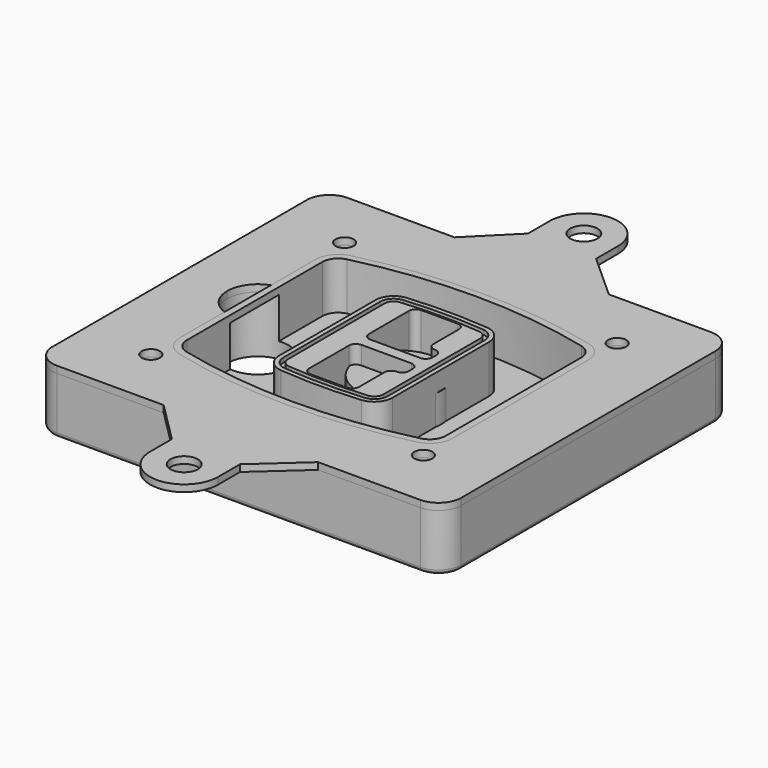
from build123d import *

# Parameters (mm, degrees)
F0_R      = 4
F1_DEPTH  = 25
F2_DEPTH  = 3
F3_DEPTH  = 18
F5_DEPTH  = 21
F6_DEPTH  = 2
F8_DEPTH  = 20
F9_DEPTH  = 16
F10_DEPTH = 25
F7_R      = 6
F7_R_2    = 4
F11_DEPTH = 6
F13_DEPTH = 9
F15_R     = 2
F16_R     = 4
F16_R_2   = 6
F17_DEPTH = 3


# Not quite as in the source:
# - a feature of the source that left no trace in its solid (it failed there, or was rolled back) is left out
# - a feature names something its author has since deleted; it is built from what else it names


with BuildPart() as f1:
    # F0 (on Top) → F1 (new body)
    with BuildSketch(Plane.XY):
        with BuildLine():
            ThreePointArc((-90, -70), (-87.0710678119, -77.0710678119), (-80, -80))
            Line((-80, -80), (80, -80))
            ThreePointArc((80, -80), (87.0710678119, -77.0710678119), (90, -70))
            Line((90, -70), (90, 70))
            ThreePointArc((90, 70), (87.0710678119, 77.0710678119), (80, 80))
            Line((80, 80), (-80, 80))
            ThreePointArc((-80, 80), (-87.0710678119, 77.0710678119), (-90, 70))
            Line((-90, 70), (-90, -70))
        make_face()
        with Locations((-60, -53.3333333333)):
            Circle(F0_R, mode=Mode.SUBTRACT)
        with Locations((60, -53.3333333333)):
            Circle(F0_R, mode=Mode.SUBTRACT)
        with Locations((-60, 53.3333333333)):
            Circle(F0_R, mode=Mode.SUBTRACT)
        with BuildLine():
            ThreePointArc((-64, 37.2990447398), (-61.0143011354, 45.9411029726), (-53.3306899286, 50.8970778549))
            ThreePointArc((-53.3306899286, 50.8970778549), (0, 57.3333333333), (53.3306899286, 50.8970778549))
            ThreePointArc((53.3306899286, 50.8970778549), (61.0143011354, 45.9411029726), (64, 37.2990447398))
            Line((64, 37.2990447398), (64, -37.2990447398))
            ThreePointArc((64, -37.2990447398), (61.0143011354, -45.9411029726), (53.3306899286, -50.8970778549))
            ThreePointArc((53.3306899286, -50.8970778549), (0, -57.3333333333), (-53.3306899286, -50.8970778549))
            ThreePointArc((-53.3306899286, -50.8970778549), (-61.0143011354, -45.9411029726), (-64, -37.2990447398))
            Line((-64, -37.2990447398), (-64, 37.2990447398))
        make_face(mode=Mode.SUBTRACT)
        with Locations((60, 53.3333333333)):
            Circle(F0_R, mode=Mode.SUBTRACT)
        with BuildLine():
            ThreePointArc((53.3306899286, 50.8970778549), (0, 57.3333333333), (-53.3306899286, 50.8970778549))
            ThreePointArc((-53.3306899286, 50.8970778549), (-61.0143011354, 45.9411029726), (-64, 37.2990447398))
            Line((-64, 37.2990447398), (-64, -37.2990447398))
            ThreePointArc((-64, -37.2990447398), (-61.0143011354, -45.9411029726), (-53.3306899286, -50.8970778549))
            ThreePointArc((-53.3306899286, -50.8970778549), (0, -57.3333333333), (53.3306899286, -50.8970778549))
            ThreePointArc((53.3306899286, -50.8970778549), (61.0143011354, -45.9411029726), (64, -37.2990447398))
            Line((64, -37.2990447398), (64, 37.2990447398))
            ThreePointArc((64, 37.2990447398), (61.0143011354, 45.9411029726), (53.3306899286, 50.8970778549))
        make_face()
        with BuildLine():
            Line((-60, -37.2990447398), (-60, 37.2990447398))
            ThreePointArc((-60, 37.2990447398), (-57.8673579538, 43.4719434775), (-52.3790642347, 47.0119255363))
            ThreePointArc((-52.3790642347, 47.0119255363), (0, 53.3333333333), (52.3790642347, 47.0119255363))
            ThreePointArc((52.3790642347, 47.0119255363), (57.8673579538, 43.4719434775), (60, 37.2990447398))
            Line((60, 37.2990447398), (60, -37.2990447398))
            ThreePointArc((60, -37.2990447398), (57.8673579538, -43.4719434775), (52.3790642347, -47.0119255363))
            ThreePointArc((52.3790642347, -47.0119255363), (0, -53.3333333333), (-52.3790642347, -47.0119255363))
            ThreePointArc((-52.3790642347, -47.0119255363), (-57.8673579538, -43.4719434775), (-60, -37.2990447398))
        make_face(mode=Mode.SUBTRACT)
        with BuildLine():
            ThreePointArc((-52.3790642347, 47.0119255363), (-57.8673579538, 43.4719434775), (-60, 37.2990447398))
            Line((-60, 37.2990447398), (-60, -37.2990447398))
            ThreePointArc((-60, -37.2990447398), (-57.8673579538, -43.4719434775), (-52.3790642347, -47.0119255363))
            ThreePointArc((-52.3790642347, -47.0119255363), (0, -53.3333333333), (52.3790642347, -47.0119255363))
            ThreePointArc((52.3790642347, -47.0119255363), (57.8673579538, -43.4719434775), (60, -37.2990447398))
            Line((60, -37.2990447398), (60, 37.2990447398))
            ThreePointArc((60, 37.2990447398), (57.8673579538, 43.4719434775), (52.3790642347, 47.0119255363))
            ThreePointArc((52.3790642347, 47.0119255363), (0, 53.3333333333), (-52.3790642347, 47.0119255363))
        make_face()
        with BuildLine():
            ThreePointArc((51.6653449643, 44.0980612973), (55.5071505677, 41.6200738562), (57, 37.2990447398))
            Line((57, 37.2990447398), (57, -37.2990447398))
            ThreePointArc((57, -37.2990447398), (55.5071505677, -41.6200738562), (51.6653449643, -44.0980612973))
            ThreePointArc((51.6653449643, -44.0980612973), (0, -50.3333333333), (-51.6653449643, -44.0980612973))
            ThreePointArc((-51.6653449643, -44.0980612973), (-55.5071505677, -41.6200738562), (-57, -37.2990447398))
            Line((-57, -37.2990447398), (-57, 37.2990447398))
            ThreePointArc((-57, 37.2990447398), (-55.5071505677, 41.6200738562), (-51.6653449643, 44.0980612973))
            ThreePointArc((-51.6653449643, 44.0980612973), (0, 50.3333333333), (51.6653449643, 44.0980612973))
        make_face(mode=Mode.SUBTRACT)
        with BuildLine():
            Line((57, -37.2990447398), (57, 37.2990447398))
            ThreePointArc((57, 37.2990447398), (55.5071505677, 41.6200738562), (51.6653449643, 44.0980612973))
            ThreePointArc((51.6653449643, 44.0980612973), (0, 50.3333333333), (-51.6653449643, 44.0980612973))
            ThreePointArc((-51.6653449643, 44.0980612973), (-55.5071505677, 41.6200738562), (-57, 37.2990447398))
            Line((-57, 37.2990447398), (-57, -37.2990447398))
            ThreePointArc((-57, -37.2990447398), (-55.5071505677, -41.6200738562), (-51.6653449643, -44.0980612973))
            ThreePointArc((-51.6653449643, -44.0980612973), (0, -50.3333333333), (51.6653449643, -44.0980612973))
            ThreePointArc((51.6653449643, -44.0980612973), (55.5071505677, -41.6200738562), (57, -37.2990447398))
        make_face()
    extrude(amount=-F1_DEPTH)

    # F0 (on Top) → F2 (join)
    with BuildSketch(Plane.XY):
        with BuildLine():
            ThreePointArc((-52.3790642347, 47.0119255363), (-57.8673579538, 43.4719434775), (-60, 37.2990447398))
            Line((-60, 37.2990447398), (-60, -37.2990447398))
            ThreePointArc((-60, -37.2990447398), (-57.8673579538, -43.4719434775), (-52.3790642347, -47.0119255363))
            ThreePointArc((-52.3790642347, -47.0119255363), (0, -53.3333333333), (52.3790642347, -47.0119255363))
            ThreePointArc((52.3790642347, -47.0119255363), (57.8673579538, -43.4719434775), (60, -37.2990447398))
            Line((60, -37.2990447398), (60, 37.2990447398))
            ThreePointArc((60, 37.2990447398), (57.8673579538, 43.4719434775), (52.3790642347, 47.0119255363))
            ThreePointArc((52.3790642347, 47.0119255363), (0, 53.3333333333), (-52.3790642347, 47.0119255363))
        make_face()
        with BuildLine():
            ThreePointArc((51.6653449643, 44.0980612973), (55.5071505677, 41.6200738562), (57, 37.2990447398))
            Line((57, 37.2990447398), (57, -37.2990447398))
            ThreePointArc((57, -37.2990447398), (55.5071505677, -41.6200738562), (51.6653449643, -44.0980612973))
            ThreePointArc((51.6653449643, -44.0980612973), (0, -50.3333333333), (-51.6653449643, -44.0980612973))
            ThreePointArc((-51.6653449643, -44.0980612973), (-55.5071505677, -41.6200738562), (-57, -37.2990447398))
            Line((-57, -37.2990447398), (-57, 37.2990447398))
            ThreePointArc((-57, 37.2990447398), (-55.5071505677, 41.6200738562), (-51.6653449643, 44.0980612973))
            ThreePointArc((-51.6653449643, 44.0980612973), (0, 50.3333333333), (51.6653449643, 44.0980612973))
        make_face(mode=Mode.SUBTRACT)
    extrude(amount=F2_DEPTH)

    # F0 (on Top) → F3 (cut)
    with BuildSketch(Plane.XY):
        with BuildLine():
            Line((57, -37.2990447398), (57, 37.2990447398))
            ThreePointArc((57, 37.2990447398), (55.5071505677, 41.6200738562), (51.6653449643, 44.0980612973))
            ThreePointArc((51.6653449643, 44.0980612973), (0, 50.3333333333), (-51.6653449643, 44.0980612973))
            ThreePointArc((-51.6653449643, 44.0980612973), (-55.5071505677, 41.6200738562), (-57, 37.2990447398))
            Line((-57, 37.2990447398), (-57, -37.2990447398))
            ThreePointArc((-57, -37.2990447398), (-55.5071505677, -41.6200738562), (-51.6653449643, -44.0980612973))
            ThreePointArc((-51.6653449643, -44.0980612973), (0, -50.3333333333), (51.6653449643, -44.0980612973))
            ThreePointArc((51.6653449643, -44.0980612973), (55.5071505677, -41.6200738562), (57, -37.2990447398))
        make_face()
    extrude(amount=-F3_DEPTH, mode=Mode.SUBTRACT)

    # F4 (on face) → F5 (join, through all)
    with BuildSketch(Plane.XY.offset(3)):
        with BuildLine():
            ThreePointArc((-25, -26.587695628), (-22.8992979869, -31.9912392117), (-17.7004291845, -34.5569740744))
            ThreePointArc((-17.7004291845, -34.5569740744), (0, -35.3333333333), (17.7004291845, -34.5569740744))
            ThreePointArc((17.7004291845, -34.5569740744), (22.8992979869, -31.9912392117), (25, -26.587695628))
            Line((25, -26.587695628), (25, 26.587695628))
            ThreePointArc((25, 26.587695628), (22.8992979869, 31.9912392117), (17.7004291845, 34.5569740744))
            ThreePointArc((17.7004291845, 34.5569740744), (0, 35.3333333333), (-17.7004291845, 34.5569740744))
            ThreePointArc((-17.7004291845, 34.5569740744), (-22.8992979869, 31.9912392117), (-25, 26.587695628))
            Line((-25, 26.587695628), (-25, -26.587695628))
        make_face()
        with BuildLine():
            ThreePointArc((17.5253218884, 32.5646544628), (21.4244734902, 30.6403533158), (23, 26.587695628))
            Line((23, 26.587695628), (23, -26.587695628))
            ThreePointArc((23, -26.587695628), (21.4244734902, -30.6403533158), (17.5253218884, -32.5646544628))
            ThreePointArc((17.5253218884, -32.5646544628), (0, -33.3333333333), (-17.5253218884, -32.5646544628))
            ThreePointArc((-17.5253218884, -32.5646544628), (-21.4244734902, -30.6403533158), (-23, -26.587695628))
            Line((-23, -26.587695628), (-23, 26.587695628))
            ThreePointArc((-23, 26.587695628), (-21.4244734902, 30.6403533158), (-17.5253218884, 32.5646544628))
            ThreePointArc((-17.5253218884, 32.5646544628), (0, 33.3333333333), (17.5253218884, 32.5646544628))
        make_face(mode=Mode.SUBTRACT)
        with BuildLine():
            Line((23, -26.587695628), (23, 26.587695628))
            ThreePointArc((23, 26.587695628), (21.4244734902, 30.6403533158), (17.5253218884, 32.5646544628))
            ThreePointArc((17.5253218884, 32.5646544628), (0, 33.3333333333), (-17.5253218884, 32.5646544628))
            ThreePointArc((-17.5253218884, 32.5646544628), (-21.4244734902, 30.6403533158), (-23, 26.587695628))
            Line((-23, 26.587695628), (-23, -26.587695628))
            ThreePointArc((-23, -26.587695628), (-21.4244734902, -30.6403533158), (-17.5253218884, -32.5646544628))
            ThreePointArc((-17.5253218884, -32.5646544628), (0, -33.3333333333), (17.5253218884, -32.5646544628))
            ThreePointArc((17.5253218884, -32.5646544628), (21.4244734902, -30.6403533158), (23, -26.587695628))
        make_face()
        with BuildLine():
            ThreePointArc((17.3502145923, 30.5723348512), (19.9496489934, 29.2894674198), (21, 26.587695628))
            Line((21, 26.587695628), (21, -26.587695628))
            ThreePointArc((21, -26.587695628), (19.9496489934, -29.2894674198), (17.3502145923, -30.5723348512))
            ThreePointArc((17.3502145923, -30.5723348512), (0, -31.3333333333), (-17.3502145923, -30.5723348512))
            ThreePointArc((-17.3502145923, -30.5723348512), (-19.9496489934, -29.2894674198), (-21, -26.587695628))
            Line((-21, -26.587695628), (-21, 26.587695628))
            ThreePointArc((-21, 26.587695628), (-19.9496489934, 29.2894674198), (-17.3502145923, 30.5723348512))
            ThreePointArc((-17.3502145923, 30.5723348512), (0, 31.3333333333), (17.3502145923, 30.5723348512))
        make_face(mode=Mode.SUBTRACT)
        with BuildLine():
            Line((21, -26.587695628), (21, 26.587695628))
            ThreePointArc((21, 26.587695628), (19.9496489934, 29.2894674198), (17.3502145923, 30.5723348512))
            ThreePointArc((17.3502145923, 30.5723348512), (0, 31.3333333333), (-17.3502145923, 30.5723348512))
            ThreePointArc((-17.3502145923, 30.5723348512), (-19.9496489934, 29.2894674198), (-21, 26.587695628))
            Line((-21, 26.587695628), (-21, -26.587695628))
            ThreePointArc((-21, -26.587695628), (-19.9496489934, -29.2894674198), (-17.3502145923, -30.5723348512))
            ThreePointArc((-17.3502145923, -30.5723348512), (0, -31.3333333333), (17.3502145923, -30.5723348512))
            ThreePointArc((17.3502145923, -30.5723348512), (19.9496489934, -29.2894674198), (21, -26.587695628))
        make_face()
        with BuildLine():
            Line((-8, -2.5), (14, -2.5))
            ThreePointArc((14, -2.5), (16.1213203436, -3.3786796564), (17, -5.5))
            Line((17, -5.5), (17, -7.5))
            ThreePointArc((17, -7.5), (16.1213203436, -9.6213203436), (14, -10.5))
            ThreePointArc((14, -10.5), (11.8786796564, -11.3786796564), (11, -13.5))
            Line((11, -13.5), (11, -27.5))
            ThreePointArc((11, -27.5), (10.1213203436, -29.6213203436), (8, -30.5))
            Line((8, -30.5), (-8, -30.5))
            ThreePointArc((-8, -30.5), (-10.1213203436, -29.6213203436), (-11, -27.5))
            Line((-11, -27.5), (-11, -5.5))
            ThreePointArc((-11, -5.5), (-10.1213203436, -3.3786796564), (-8, -2.5))
        make_face(mode=Mode.SUBTRACT)
        with BuildLine():
            ThreePointArc((-8, 2.5), (-10.1213203436, 3.3786796564), (-11, 5.5))
            Line((-11, 5.5), (-11, 27.5))
            ThreePointArc((-11, 27.5), (-10.1213203436, 29.6213203436), (-8, 30.5))
            Line((-8, 30.5), (8, 30.5))
            ThreePointArc((8, 30.5), (10.1213203436, 29.6213203436), (11, 27.5))
            Line((11, 27.5), (11, 13.5))
            ThreePointArc((11, 13.5), (11.8786796564, 11.3786796564), (14, 10.5))
            ThreePointArc((14, 10.5), (16.1213203436, 9.6213203436), (17, 7.5))
            Line((17, 7.5), (17, 5.5))
            ThreePointArc((17, 5.5), (16.1213203436, 3.3786796564), (14, 2.5))
            Line((14, 2.5), (-8, 2.5))
        make_face(mode=Mode.SUBTRACT)
    extrude(amount=-F5_DEPTH)

    # F4 (on face) → F6 (cut)
    with BuildSketch(Plane.XY.offset(3)):
        with BuildLine():
            Line((23, -26.587695628), (23, 26.587695628))
            ThreePointArc((23, 26.587695628), (21.4244734902, 30.6403533158), (17.5253218884, 32.5646544628))
            ThreePointArc((17.5253218884, 32.5646544628), (0, 33.3333333333), (-17.5253218884, 32.5646544628))
            ThreePointArc((-17.5253218884, 32.5646544628), (-21.4244734902, 30.6403533158), (-23, 26.587695628))
            Line((-23, 26.587695628), (-23, -26.587695628))
            ThreePointArc((-23, -26.587695628), (-21.4244734902, -30.6403533158), (-17.5253218884, -32.5646544628))
            ThreePointArc((-17.5253218884, -32.5646544628), (0, -33.3333333333), (17.5253218884, -32.5646544628))
            ThreePointArc((17.5253218884, -32.5646544628), (21.4244734902, -30.6403533158), (23, -26.587695628))
        make_face()
        with BuildLine():
            ThreePointArc((17.3502145923, 30.5723348512), (19.9496489934, 29.2894674198), (21, 26.587695628))
            Line((21, 26.587695628), (21, -26.587695628))
            ThreePointArc((21, -26.587695628), (19.9496489934, -29.2894674198), (17.3502145923, -30.5723348512))
            ThreePointArc((17.3502145923, -30.5723348512), (0, -31.3333333333), (-17.3502145923, -30.5723348512))
            ThreePointArc((-17.3502145923, -30.5723348512), (-19.9496489934, -29.2894674198), (-21, -26.587695628))
            Line((-21, -26.587695628), (-21, 26.587695628))
            ThreePointArc((-21, 26.587695628), (-19.9496489934, 29.2894674198), (-17.3502145923, 30.5723348512))
            ThreePointArc((-17.3502145923, 30.5723348512), (0, 31.3333333333), (17.3502145923, 30.5723348512))
        make_face(mode=Mode.SUBTRACT)
    extrude(amount=-F6_DEPTH, mode=Mode.SUBTRACT)

    # F7 (on face) → F8 (join)
    with BuildSketch(Plane(origin=(0, 0, -25), x_dir=(1, 0, 0), z_dir=(0, 0, -1))):
        with BuildLine():
            ThreePointArc((-6.71157564, 0), (6.7567035675, 13.4682792075), (20.224982775, 0))
            Line((20.224982775, 0), (25.224982775, 0))
            ThreePointArc((25.224982775, 0), (6.7567035675, 18.4682792075), (-11.71157564, 0))
            Line((-11.71157564, 0), (-6.71157564, 0))
        make_face()
        with BuildLine():
            Line((-6.71157564, 0), (20.224982775, 0))
            ThreePointArc((20.224982775, 0), (6.7567035675, 13.4682792075), (-6.71157564, 0))
        make_face()
        with BuildLine():
            ThreePointArc((-6.71157564, 0), (6.7567035675, -13.4682792075), (20.224982775, 0))
            Line((20.224982775, 0), (-6.71157564, 0))
        make_face()
        with BuildLine():
            Line((25.224982775, 0), (20.224982775, 0))
            ThreePointArc((20.224982775, 0), (6.7567035675, -13.4682792075), (-6.71157564, 0))
            Line((-6.71157564, 0), (-11.71157564, 0))
            ThreePointArc((-11.71157564, 0), (6.7567035675, -18.4682792075), (25.224982775, 0))
        make_face()
    extrude(amount=-F8_DEPTH)

    # F7 (on face) → F9 (cut)
    with BuildSketch(Plane(origin=(0, 0, -25), x_dir=(1, 0, 0), z_dir=(0, 0, -1))):
        with BuildLine():
            Line((-6.71157564, 0), (20.224982775, 0))
            ThreePointArc((20.224982775, 0), (6.7567035675, 13.4682792075), (-6.71157564, 0))
        make_face()
        with BuildLine():
            ThreePointArc((-6.71157564, 0), (6.7567035675, -13.4682792075), (20.224982775, 0))
            Line((20.224982775, 0), (-6.71157564, 0))
        make_face()
    extrude(amount=-F9_DEPTH, mode=Mode.SUBTRACT)

    # F7 (on face) → F10 (cut)
    with BuildSketch(Plane(origin=(0, 0, -25), x_dir=(1, 0, 0), z_dir=(0, 0, -1))):
        with BuildLine():
            Line((-69.0318229325, 0), (-42.0952645175, 0))
            ThreePointArc((-42.0952645175, 0), (-55.563543725, 13.4682792075), (-69.0318229325, 0))
        make_face()
        with BuildLine():
            ThreePointArc((-69.0318229325, 0), (-55.563543725, -13.4682792075), (-42.0952645175, 0))
            Line((-42.0952645175, 0), (-69.0318229325, 0))
        make_face()
    extrude(amount=-F10_DEPTH, mode=Mode.SUBTRACT)

    # F7 (on face) → F11 (cut)
    with BuildSketch(Plane(origin=(0, 0, -25), x_dir=(1, 0, 0), z_dir=(0, 0, -1))):
        with Locations((60, -53.3333333333)):
            Circle(F7_R)
        with Locations((60, -53.3333333333)):
            Circle(F7_R_2, mode=Mode.SUBTRACT)
        with Locations((-60, -53.3333333333)):
            Circle(F7_R)
        with Locations((-60, -53.3333333333)):
            Circle(F7_R_2, mode=Mode.SUBTRACT)
        with Locations((-60, 53.3333333333)):
            Circle(F7_R)
        with Locations((-60, 53.3333333333)):
            Circle(F7_R_2, mode=Mode.SUBTRACT)
        with Locations((60, 53.3333333333)):
            Circle(F7_R)
        with Locations((60, 53.3333333333)):
            Circle(F7_R_2, mode=Mode.SUBTRACT)
    extrude(amount=-F11_DEPTH, mode=Mode.SUBTRACT)

    # F12 (on face) → F13 (cut, through all)
    with BuildSketch(Plane(origin=(0, 0, -9), x_dir=(1, 0, 0), z_dir=(0, 0, -1))):
        with BuildLine():
            ThreePointArc((20.224982775, 0), (20.1663399806, 1.2554664788), (19.9909222755, 2.5))
            Line((19.9909222755, 2.5), (14, 2.5))
            ThreePointArc((14, 2.5), (16.1213203436, 3.3786796564), (17, 5.5))
            Line((17, 5.5), (17, 7.5))
            ThreePointArc((17, 7.5), (16.1213203436, 9.6213203436), (14, 10.5))
            ThreePointArc((14, 10.5), (12.1627255951, 11.1284134507), (11.0951631559, 12.750384826))
            ThreePointArc((11.0951631559, 12.750384826), (11.0476113807, 12.7664660322), (11, 12.7823698976))
            Line((11, 12.7823698976), (11, -12.7823698976))
            ThreePointArc((11, -12.7823698976), (11.0476113807, -12.7664660322), (11.0951631559, -12.750384826))
            ThreePointArc((11.0951631559, -12.750384826), (12.1627255951, -11.1284134507), (14, -10.5))
            ThreePointArc((14, -10.5), (16.1213203436, -9.6213203436), (17, -7.5))
            Line((17, -7.5), (17, -5.5))
            ThreePointArc((17, -5.5), (16.1213203436, -3.3786796564), (14, -2.5))
            Line((14, -2.5), (19.9909222755, -2.5))
            ThreePointArc((19.9909222755, -2.5), (20.1663399806, -1.2554664788), (20.224982775, 0))
        make_face()
    extrude(amount=F13_DEPTH, mode=Mode.SUBTRACT)

    # F15
    f15_edges = [f1.edges().sort_by_distance(p)[0] for p in [
        (0, -80, -25),
        (-87.071068, -77.071068, -25),
        (-90, 0, -25),
        (-87.071068, 77.071068, -25),
        (87.071068, -77.071068, -25),
        (0, 80, -25),
        (90, 0, -25),
        (87.071068, 77.071068, -25),
    ]]
    fillet(f15_edges, radius=F15_R)


with BuildPart() as f17:
    # F16 (on face) → F17 (new body, through all)
    with BuildSketch(Plane.XY):
        with BuildLine():
            Line((35, 80), (-33, 80))
            Line((-33, 80), (-80, 80))
            ThreePointArc((-80, 80), (-87.0710678119, 77.0710678119), (-90, 70))
            Line((-90, 70), (-90, -70))
            ThreePointArc((-90, -70), (-87.0710678119, -77.0710678119), (-80, -80))
            Line((-80, -80), (-33, -80))
            Line((-33, -80), (35, -80))
            Line((35, -80), (80, -80))
            ThreePointArc((80, -80), (87.0710678119, -77.0710678119), (90, -70))
            Line((90, -70), (90, 70))
            ThreePointArc((90, 70), (87.0710678119, 77.0710678119), (80, 80))
            Line((80, 80), (35, 80))
        make_face()
        with Locations((-60, -53.3333333333)):
            Circle(F16_R, mode=Mode.SUBTRACT)
        with Locations((60, -53.3333333333)):
            Circle(F16_R, mode=Mode.SUBTRACT)
        with Locations((-60, 53.3333333333)):
            Circle(F16_R, mode=Mode.SUBTRACT)
        with BuildLine():
            Line((-60, 12.7166190685), (-60, 37.2990447398))
            ThreePointArc((-60, 37.2990447398), (-57.8673579538, 43.4719434775), (-52.3790642347, 47.0119255363))
            ThreePointArc((-52.3790642347, 47.0119255363), (0, 53.3333333333), (52.3790642347, 47.0119255363))
            ThreePointArc((52.3790642347, 47.0119255363), (57.8673579538, 43.4719434775), (60, 37.2990447398))
            Line((60, 37.2990447398), (60, -37.2990447398))
            ThreePointArc((60, -37.2990447398), (57.8673579538, -43.4719434775), (52.3790642347, -47.0119255363))
            ThreePointArc((52.3790642347, -47.0119255363), (0, -53.3333333333), (-52.3790642347, -47.0119255363))
            ThreePointArc((-52.3790642347, -47.0119255363), (-57.8673579538, -43.4719434775), (-60, -37.2990447398))
            Line((-60, -37.2990447398), (-60, -12.7166190685))
            ThreePointArc((-60, -12.7166190685), (-66.5441169481, -7.798817635), (-69.0318229325, 0))
            ThreePointArc((-69.0318229325, 0), (-66.5441169481, 7.798817635), (-60, 12.7166190685))
        make_face(mode=Mode.SUBTRACT)
        with Locations((60, 53.3333333333)):
            Circle(F16_R, mode=Mode.SUBTRACT)
        with BuildLine():
            Line((-15, 98), (-33, 80))
            Line((-33, 80), (35, 80))
            Line((35, 80), (15, 98))
            Line((15, 98), (15, 110))
            ThreePointArc((15, 110), (0, 125), (-15, 110))
            Line((-15, 110), (-15, 98))
        make_face()
        with Locations((0, 110)):
            Circle(F16_R_2, mode=Mode.SUBTRACT)
        with BuildLine():
            Line((35, -80), (-33, -80))
            Line((-33, -80), (-15, -98))
            Line((-15, -98), (-15, -110))
            ThreePointArc((-15, -110), (0, -125), (15, -110))
            Line((15, -110), (15, -98))
            Line((15, -98), (35, -80))
        make_face()
        with Locations((0, -110)):
            Circle(F16_R_2, mode=Mode.SUBTRACT)
    extrude(amount=F17_DEPTH)


solid = Compound([f1.part, f17.part])
